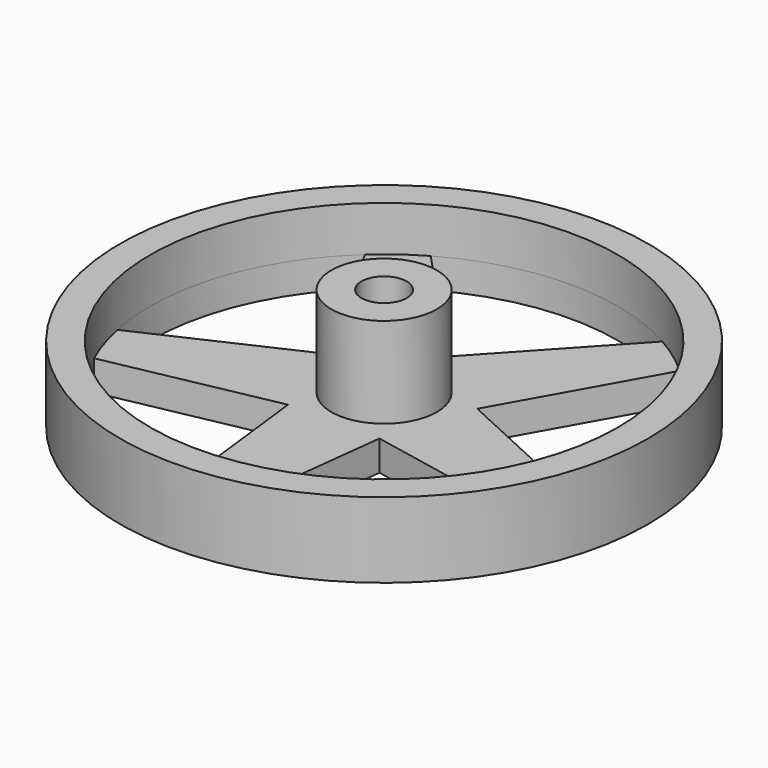
from build123d import *

# Parameters (mm, degrees)
F0_R     = 17.5
F1_DEPTH = 5
F2_R     = 15.5
F3_DEPTH = 3
F4_R     = 3.5
F4_R_2   = 1.5
F5_DEPTH = 6
F7_DEPTH = 1
F8_DEPTH = 2


with BuildPart() as f1:
    # F0 (on Top) → F1 (new body)
    with BuildSketch(Plane.XY):
        Circle(F0_R)
    extrude(amount=F1_DEPTH)

    # F2 (on face) → F3 (cut)
    with BuildSketch(Plane.XY.offset(5)):
        Circle(F2_R)
    extrude(amount=-F3_DEPTH, mode=Mode.SUBTRACT)

    # F4 (on face) → F5 (join)
    with BuildSketch(Plane.XY.offset(2)):
        Circle(F4_R)
        Circle(F4_R_2, mode=Mode.SUBTRACT)
    extrude(amount=F5_DEPTH)

    # F6 (on face) → F7 (cut)
    with BuildSketch(Plane(origin=(0, 0, 0), x_dir=(1, 0, 0), z_dir=(0, 0, -1))):
        Polygon((-3.9243327608, 0.1564746204), (-3.3940706843, 1.1028004157), (-3.2668253693, 2.1800742948), (-12.161596097, 3.9515421095), align=None)
        Polygon((1.0638693073, 3.7806155611), (0, 12.7874588824), (-1.0638693073, 3.7806155611), (0, 3.5687371109), align=None)
        Polygon((3.2668253693, 2.1800742948), (3.3940706843, 1.1028004157), (3.9243327608, 0.1564746204), (12.161596097, 3.9515421095), align=None)
        Polygon((3.0828784209, -2.4332555489), (2.0976510431, -2.8871689712), (1.361501722, -3.6839089274), (7.5162797454, -10.3452715508), align=None)
        Polygon((-1.361501722, -3.6839089274), (-2.0976510431, -2.8871689712), (-3.0828784209, -2.4332555489), (-7.5162797454, -10.3452715508), align=None)
    extrude(amount=-F7_DEPTH, mode=Mode.SUBTRACT)

    # F6 (on face) → F8 (cut)
    with BuildSketch(Plane(origin=(0, 0, 0), x_dir=(1, 0, 0), z_dir=(0, 0, -1))):
        with BuildLine():
            Line((7.6763518896, -13.4656459803), (0, -5.1574724983))
            Line((0, -5.1574724983), (-7.6763518896, -13.4656459803))
            ThreePointArc((-7.6763518896, -13.4656459803), (0, -15.5), (7.6763518896, -13.4656459803))
        make_face()
        with BuildLine():
            Line((-10.434467167, -11.4617579341), (-4.9050478272, -1.59374665))
            Line((-4.9050478272, -1.59374665), (-15.1787135444, 3.1395310378))
            ThreePointArc((-15.1787135444, 3.1395310378), (-14.7413760026, -4.7897634128), (-10.434467167, -11.4617579341))
        make_face()
        with BuildLine():
            Line((1.7046089863, 15.4059828704), (3.0314862736, 4.1724828992))
            Line((3.0314862736, 4.1724828992), (14.1252072533, 6.3818900062))
            ThreePointArc((14.1252072533, 6.3818900062), (9.1106714105, 12.5397634128), (1.7046089863, 15.4059828704))
        make_face()
        with BuildLine():
            Line((15.1787135444, 3.1395310378), (4.9050478272, -1.59374665))
            Line((4.9050478272, -1.59374665), (10.434467167, -11.4617579341))
            ThreePointArc((10.434467167, -11.4617579341), (14.1771689891, -6.2656108605), (15.5, 0))
            ThreePointArc((15.5, 0), (15.4194691857, 1.5779638877), (15.1787135444, 3.1395310378))
        make_face()
        with BuildLine():
            Line((-14.1252072533, 6.3818900062), (-3.0314862736, 4.1724828992))
            Line((-3.0314862736, 4.1724828992), (-1.7046089863, 15.4059828704))
            ThreePointArc((-1.7046089863, 15.4059828704), (-9.1106714105, 12.5397634128), (-14.1252072533, 6.3818900062))
        make_face()
    extrude(amount=-F8_DEPTH, mode=Mode.SUBTRACT)


solid = f1.part
